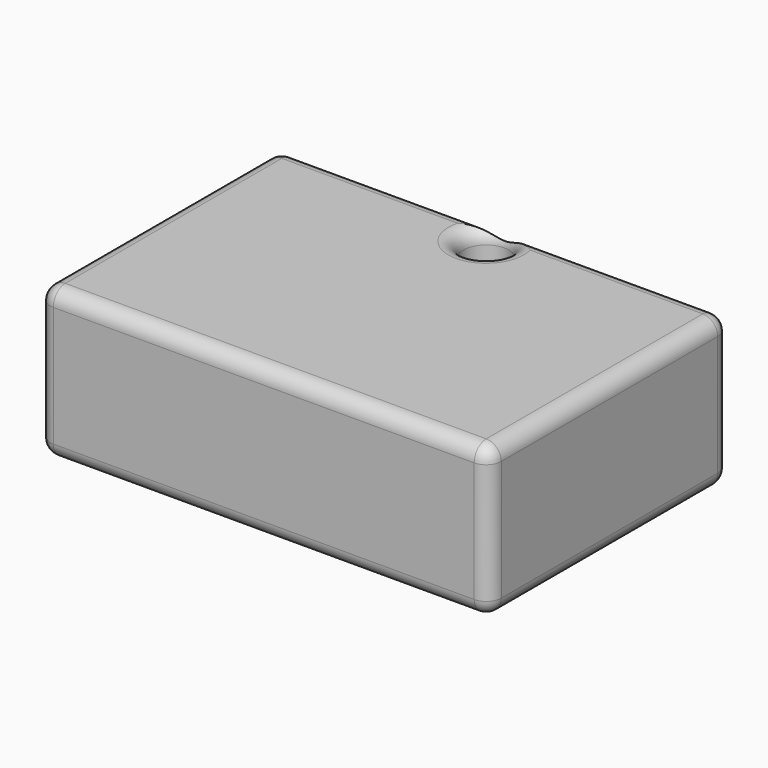
from build123d import *

# Parameters (mm, degrees)
F0_W         = 300
F0_H         = 200
F0_R         = 15
F1_DEPTH     = 100
F2_R         = 10
F3_R         = 10
F4_R         = 10
F5_R         = 10
F6_T1_DEPTH  = 280
F6_T3_DEPTH  = 180
F6_T6_ANGLE  = 90
F6_T8_ANGLE  = 90
F6_T10_ANGLE = 90
F6_T12_ANGLE = 90
F7_T1_DEPTH  = 280
F7_T3_DEPTH  = 180
F7_T6_ANGLE  = 90
F7_T8_ANGLE  = 90
F7_T10_ANGLE = 90
F7_T12_ANGLE = 90


# Not quite as in the source:
# - a fillet or chamfer that OpenCascade refuses, or shapes differently, is made with other operations: its cross-section is extruded or revolved along the edge and cut away or added


with BuildPart() as f1:
    # F0 (on Top) → F1 (new body)
    with BuildSketch(Plane.XY):
        with Locations((-0.982619822, 16.5327907399)):
            Rectangle(F0_W, F0_H)
        with Locations((0, 100.119560957)):
            Circle(F0_R, mode=Mode.SUBTRACT)
    extrude(amount=F1_DEPTH)

    # F2
    f2_edges = [f1.edges().sort_by_distance(p)[0] for p in [
        (149.01738, 116.532791, 50),
    ]]
    fillet(f2_edges, radius=F2_R)

    # F3
    f3_edges = [f1.edges().sort_by_distance(p)[0] for p in [
        (-150.98262, 116.532791, 50),
    ]]
    fillet(f3_edges, radius=F3_R)

    # F4
    f4_edges = [f1.edges().sort_by_distance(p)[0] for p in [
        (149.01738, -83.467209, 50),
    ]]
    fillet(f4_edges, radius=F4_R)

    # F5
    f5_edges = [f1.edges().sort_by_distance(p)[0] for p in [
        (-150.98262, -83.467209, 50),
    ]]
    fillet(f5_edges, radius=F5_R)

    # F6: fillet of radius 10 on 9 edges, made by hand

    # F6_s2 → F6_t1 (cut)
    with BuildSketch(Plane.YZ.offset(-140.982619822)):
        with BuildLine():
            ThreePointArc((-83.4672092601, 90), (-80.538277072, 97.0710678119), (-73.4672092601, 100))
            Line((-73.4672092601, 100), (-83.4672092601, 100))
            Line((-83.4672092601, 100), (-83.4672092601, 90))
        make_face()
        with BuildLine():
            ThreePointArc((116.5327907399, 90), (113.6038585518, 97.0710678119), (106.5327907399, 100))
            Line((106.5327907399, 100), (116.5327907399, 100))
            Line((116.5327907399, 100), (116.5327907399, 90))
        make_face()
    extrude(amount=F6_T1_DEPTH, mode=Mode.SUBTRACT)

    # F6_s4 → F6_t3 (cut)
    with BuildSketch(Plane.XZ.offset(-106.5327907399)):
        with BuildLine():
            ThreePointArc((-150.982619822, 90), (-148.0536876339, 97.0710678119), (-140.982619822, 100))
            Line((-140.982619822, 100), (-150.982619822, 100))
            Line((-150.982619822, 100), (-150.982619822, 90))
        make_face()
        with BuildLine():
            ThreePointArc((149.017380178, 90), (146.0884479898, 97.0710678119), (139.017380178, 100))
            Line((139.017380178, 100), (149.017380178, 100))
            Line((149.017380178, 100), (149.017380178, 90))
        make_face()
    extrude(amount=F6_T3_DEPTH, mode=Mode.SUBTRACT)

    # F6_s5 → F6_t6 (revolve, cut)
    with BuildSketch(Plane.YZ.offset(-140.982619822)):
        with BuildLine():
            ThreePointArc((-83.4672092601, 90), (-80.538277072, 97.0710678119), (-73.4672092601, 100))
            Line((-73.4672092601, 100), (-83.4672092601, 100))
            Line((-83.4672092601, 100), (-83.4672092601, 90))
        make_face()
    revolve(axis=Axis((-140.982619822, -73.4672092601, 100), (0, 0, -1)), revolution_arc=F6_T6_ANGLE, mode=Mode.SUBTRACT)

    # F6_s7 → F6_t8 (revolve, cut)
    with BuildSketch(Plane.XZ.offset(73.4672092601)):
        with BuildLine():
            ThreePointArc((149.017380178, 90), (146.0884479898, 97.0710678119), (139.017380178, 100))
            Line((139.017380178, 100), (149.017380178, 100))
            Line((149.017380178, 100), (149.017380178, 90))
        make_face()
    revolve(axis=Axis((139.017380178, -73.4672092601, 100), (0, 0, -1)), revolution_arc=F6_T8_ANGLE, mode=Mode.SUBTRACT)

    # F6_s9 → F6_t10 (revolve, cut)
    with BuildSketch(Plane.YZ.offset(-140.982619822)):
        with BuildLine():
            ThreePointArc((116.5327907399, 90), (113.6038585518, 97.0710678119), (106.5327907399, 100))
            Line((106.5327907399, 100), (116.5327907399, 100))
            Line((116.5327907399, 100), (116.5327907399, 90))
        make_face()
    revolve(axis=Axis((-140.982619822, 106.5327907399, 100), (0, 0, 1)), revolution_arc=F6_T10_ANGLE, mode=Mode.SUBTRACT)

    # F6_s11 → F6_t12 (revolve, cut)
    with BuildSketch(Plane.XZ.offset(-106.5327907399)):
        with BuildLine():
            ThreePointArc((149.017380178, 90), (146.0884479898, 97.0710678119), (139.017380178, 100))
            Line((139.017380178, 100), (149.017380178, 100))
            Line((149.017380178, 100), (149.017380178, 90))
        make_face()
    revolve(axis=Axis((139.017380178, 106.5327907399, 100), (0, 0, 1)), revolution_arc=F6_T12_ANGLE, mode=Mode.SUBTRACT)

    # F6_s13 → F6_t14 (revolve, cut)
    with BuildSketch(Plane.XZ.offset(-100.119560957)):
        with BuildLine():
            ThreePointArc((15, 90), (17.9289321881, 97.0710678119), (25, 100))
            Line((25, 100), (15, 100))
            Line((15, 100), (15, 90))
        make_face()
    revolve(axis=Axis((0, 100.119560957, 100), (0, 0, 1)), mode=Mode.SUBTRACT)

    # F7: fillet of radius 10 on 9 edges, made by hand

    # F7_s2 → F7_t1 (cut)
    with BuildSketch(Plane.YZ.offset(-140.982619822)):
        with BuildLine():
            ThreePointArc((-73.4672092601, 0), (-80.538277072, 2.9289321881), (-83.4672092601, 10))
            Line((-83.4672092601, 10), (-83.4672092601, 0))
            Line((-83.4672092601, 0), (-73.4672092601, 0))
        make_face()
        with BuildLine():
            ThreePointArc((106.5327907399, 0), (113.6038585518, 2.9289321881), (116.5327907399, 10))
            Line((116.5327907399, 10), (116.5327907399, 0))
            Line((116.5327907399, 0), (106.5327907399, 0))
        make_face()
    extrude(amount=F7_T1_DEPTH, mode=Mode.SUBTRACT)

    # F7_s4 → F7_t3 (cut)
    with BuildSketch(Plane.XZ.offset(-106.5327907399)):
        with BuildLine():
            ThreePointArc((-140.982619822, 0), (-148.0536876339, 2.9289321881), (-150.982619822, 10))
            Line((-150.982619822, 10), (-150.982619822, 0))
            Line((-150.982619822, 0), (-140.982619822, 0))
        make_face()
        with BuildLine():
            ThreePointArc((139.017380178, 0), (146.0884479898, 2.9289321881), (149.017380178, 10))
            Line((149.017380178, 10), (149.017380178, 0))
            Line((149.017380178, 0), (139.017380178, 0))
        make_face()
    extrude(amount=F7_T3_DEPTH, mode=Mode.SUBTRACT)

    # F7_s5 → F7_t6 (revolve, cut)
    with BuildSketch(Plane.YZ.offset(-140.982619822)):
        with BuildLine():
            ThreePointArc((-73.4672092601, 0), (-80.538277072, 2.9289321881), (-83.4672092601, 10))
            Line((-83.4672092601, 10), (-83.4672092601, 0))
            Line((-83.4672092601, 0), (-73.4672092601, 0))
        make_face()
    revolve(axis=Axis((-140.982619822, -73.4672092601, 0), (0, 0, -1)), revolution_arc=F7_T6_ANGLE, mode=Mode.SUBTRACT)

    # F7_s7 → F7_t8 (revolve, cut)
    with BuildSketch(Plane.XZ.offset(73.4672092601)):
        with BuildLine():
            ThreePointArc((139.017380178, 0), (146.0884479898, 2.9289321881), (149.017380178, 10))
            Line((149.017380178, 10), (149.017380178, 0))
            Line((149.017380178, 0), (139.017380178, 0))
        make_face()
    revolve(axis=Axis((139.017380178, -73.4672092601, 0), (0, 0, -1)), revolution_arc=F7_T8_ANGLE, mode=Mode.SUBTRACT)

    # F7_s9 → F7_t10 (revolve, cut)
    with BuildSketch(Plane.YZ.offset(-140.982619822)):
        with BuildLine():
            ThreePointArc((106.5327907399, 0), (113.6038585518, 2.9289321881), (116.5327907399, 10))
            Line((116.5327907399, 10), (116.5327907399, 0))
            Line((116.5327907399, 0), (106.5327907399, 0))
        make_face()
    revolve(axis=Axis((-140.982619822, 106.5327907399, 0), (0, 0, 1)), revolution_arc=F7_T10_ANGLE, mode=Mode.SUBTRACT)

    # F7_s11 → F7_t12 (revolve, cut)
    with BuildSketch(Plane.XZ.offset(-106.5327907399)):
        with BuildLine():
            ThreePointArc((139.017380178, 0), (146.0884479898, 2.9289321881), (149.017380178, 10))
            Line((149.017380178, 10), (149.017380178, 0))
            Line((149.017380178, 0), (139.017380178, 0))
        make_face()
    revolve(axis=Axis((139.017380178, 106.5327907399, 0), (0, 0, 1)), revolution_arc=F7_T12_ANGLE, mode=Mode.SUBTRACT)

    # F7_s13 → F7_t14 (revolve, cut)
    with BuildSketch(Plane.XZ.offset(-100.119560957)):
        with BuildLine():
            ThreePointArc((25, 0), (17.9289321881, 2.9289321881), (15, 10))
            Line((15, 10), (15, 0))
            Line((15, 0), (25, 0))
        make_face()
    revolve(axis=Axis((0, 100.119560957, 0), (0, 0, 1)), mode=Mode.SUBTRACT)


solid = f1.part
